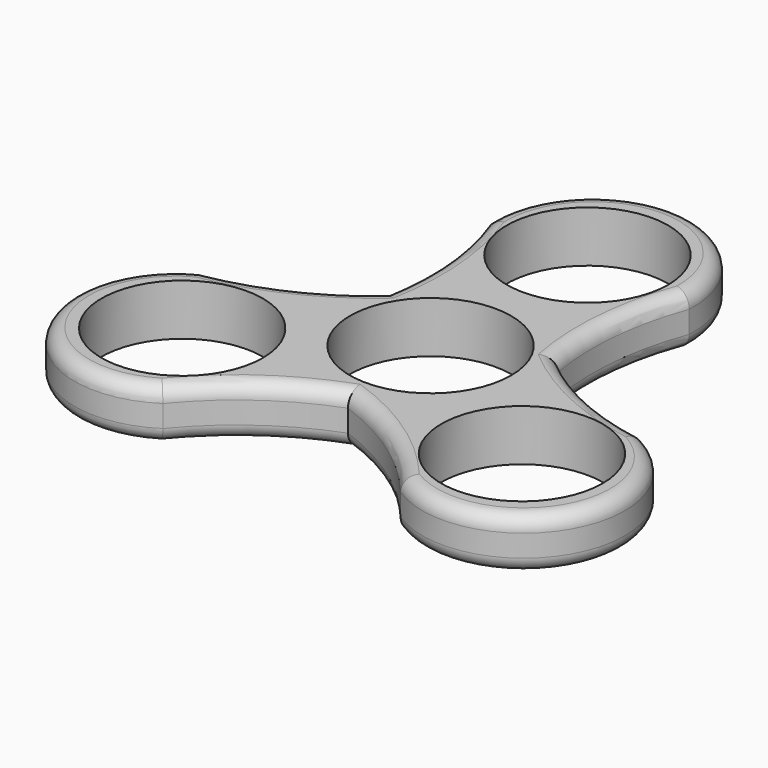
from build123d import *

# Parameters (mm, degrees)
F0_R         = 11
F1_DEPTH     = 7
F2_T3_ANGLE  = 45.2058743493
F2_S4_R      = 38
F2_T5_DEPTH  = 19
F2_T8_ANGLE  = 227.522654694
F2_T11_ANGLE = 45.8937746322
F2_S12_R     = 38
F2_T13_DEPTH = 20
F2_T16_ANGLE = 45.2058743493
F2_S17_R     = 38
F2_T18_DEPTH = 20
F2_T21_ANGLE = 227.522654694
F2_T24_ANGLE = 45.8937746322
F2_S25_R     = 38
F2_T26_DEPTH = 21
F2_T29_ANGLE = 45.2058743493
F2_S30_R     = 38
F2_T31_DEPTH = 21
F2_T34_ANGLE = 227.522654694
F2_T37_ANGLE = 45.8937746322
F2_S38_R     = 38
F2_T39_DEPTH = 20
F2_T43_ANGLE = 45.2058743493
F2_S44_R     = 38
F2_T45_DEPTH = 19
F2_T48_ANGLE = 45.8937746322
F2_S49_R     = 38
F2_T50_DEPTH = 20
F2_T55_ANGLE = 45.8937746322
F2_S56_R     = 38
F2_T57_DEPTH = 20
F2_T60_ANGLE = 45.2058743493
F2_S61_R     = 38
F2_T62_DEPTH = 20
F2_T67_ANGLE = 45.2058743493
F2_S68_R     = 38
F2_T69_DEPTH = 21
F2_T72_ANGLE = 45.8937746322
F2_S73_R     = 38
F2_T74_DEPTH = 21
F3_T3_ANGLE  = 227.522654694
F3_T6_ANGLE  = 45.2058743493
F3_S7_R      = 38
F3_T8_DEPTH  = 19
F3_T11_ANGLE = 45.8937746322
F3_S12_R     = 38
F3_T13_DEPTH = 20
F3_T16_ANGLE = 227.522654694
F3_T19_ANGLE = 45.2058743493
F3_S20_R     = 38
F3_T21_DEPTH = 21
F3_T24_ANGLE = 45.8937746322
F3_S25_R     = 38
F3_T26_DEPTH = 21
F3_T29_ANGLE = 227.522654694
F3_T32_ANGLE = 45.2058743493
F3_S33_R     = 38
F3_T34_DEPTH = 20
F3_T37_ANGLE = 45.8937746322
F3_S38_R     = 38
F3_T39_DEPTH = 20
F3_T43_ANGLE = 45.8937746322
F3_S44_R     = 38
F3_T45_DEPTH = 20
F3_T48_ANGLE = 45.2058743493
F3_S49_R     = 38
F3_T50_DEPTH = 19
F3_T55_ANGLE = 45.8937746322
F3_S56_R     = 38
F3_T57_DEPTH = 21
F3_T60_ANGLE = 45.2058743493
F3_S61_R     = 38
F3_T62_DEPTH = 21
F3_T67_ANGLE = 45.8937746322
F3_S68_R     = 38
F3_T69_DEPTH = 20
F3_T72_ANGLE = 45.2058743493
F3_S73_R     = 38
F3_T74_DEPTH = 20


# Not quite as in the source:
# - a fillet or chamfer that OpenCascade refuses, or shapes differently, is made with other operations: its cross-section is extruded or revolved along the edge and cut away or added


with BuildPart() as f1:
    # F0 (on Top) → F1 (new body)
    with BuildSketch(Plane.XY):
        with BuildLine():
            ThreePointArc((12.0468410067, 6.6555924166), (11.6038749685, 16.833912258), (13.8810481876, 26.764113456))
            ThreePointArc((13.8810481876, 26.764113456), (0.0907252543, 41.2909770134), (-13.6995976791, 26.764113456))
            ThreePointArc((-13.6995976791, 26.764113456), (-11.4438268991, 17.0610116136), (-11.7873326133, 7.1050741388))
            ThreePointArc((-11.7873326133, 7.1050741388), (-20.3805331447, 1.6322943761), (-30.1189262565, -1.3607163664))
            ThreePointArc((-30.1189262565, -1.3607163664), (-35.8043976678, -20.5669181317), (-16.3286033231, -25.2462563397))
            ThreePointArc((-16.3286033231, -25.2462563397), (-9.053356022, -18.4411506179), (-0.2595083933, -13.7606665554))
            ThreePointArc((-0.2595083933, -13.7606665554), (8.7766581762, -18.466206634), (16.2378780689, -25.4033970896))
            ThreePointArc((16.2378780689, -25.4033970896), (35.7136724135, -20.7240588817), (30.0282010022, -1.5178571163))
            ThreePointArc((30.0282010022, -1.5178571163), (20.4971829212, 1.3801390044), (12.0468410067, 6.6555924166))
        make_face()
        with Locations((-23.1784021627, -13.382056728)):
            Circle(F0_R, mode=Mode.SUBTRACT)
        with Locations((23.1784021627, -13.382056728)):
            Circle(F0_R, mode=Mode.SUBTRACT)
        Circle(F0_R, mode=Mode.SUBTRACT)
        with Locations((0, 26.764113456)):
            Circle(F0_R, mode=Mode.SUBTRACT)
    extrude(amount=F1_DEPTH)

    # F2: fillet of radius 2 on 9 edges, made by hand


with BuildPart() as f2_tool1:
    # F2_s2 → F2_t3 (revolve)
    with BuildSketch(Plane(origin=(-16.5393520653, 30.8992120032, 0), x_dir=(0, 0, 1), z_dir=(-0.4719154962, 0.8816437855, 0))):
        with BuildLine():
            ThreePointArc((5, 0.8807372995), (6.4142135624, 1.4665237371), (7, 2.8807372995))
            Line((7, 2.8807372995), (7, 0.8807372995))
            Line((7, 0.8807372995), (5, 0.8807372995))
        make_face()
    revolve(axis=Axis((-49.2653193466, 13.382056728, 7), (0, 0, -1)), revolution_arc=F2_T3_ANGLE)

    # F2_s4 → F2_t5 (intersect, symmetric)
    with BuildSketch(Plane.XY.offset(5.3)):
        with Locations((-36.3125860089, 36.1311304656)):
            Circle(F2_S4_R)
    extrude(amount=F2_T5_DEPTH, both=True, mode=Mode.INTERSECT)


with BuildPart() as f2_tool6:
    # F2_s7 → F2_t8 (revolve)
    with BuildSketch(Plane(origin=(10.1493203818, 23.0537204739, 0), x_dir=(0, 0, 1), z_dir=(-0.4029276386, -0.9152318384, 0))):
        with BuildLine():
            ThreePointArc((5, -2.8187794742), (6.4142135624, -2.2329930365), (7, -0.8187794742))
            Line((7, -0.8187794742), (7, -2.8187794742))
            Line((7, -2.8187794742), (5, -2.8187794742))
        make_face()
    revolve(axis=Axis((0.0907252543, 27.4819820491, 7), (0, 0, 1)), revolution_arc=F2_T8_ANGLE)


with BuildPart() as f2_tool9:
    # F2_s10 → F2_t11 (revolve)
    with BuildSketch(Plane(origin=(0.7055478119, -2.2061129258, 0), x_dir=(0, 0, 1), z_dir=(0.3046158068, -0.9524753069, 0))):
        with BuildLine():
            ThreePointArc((5, -13.1732132997), (6.4142135624, -12.5874268621), (7, -11.1732132997))
            Line((7, -11.1732132997), (7, -13.1732132997))
            Line((7, -13.1732132997), (5, -13.1732132997))
        make_face()
    revolve(axis=Axis((49.4467698551, 13.382056728, 7), (0, 0, -1)), revolution_arc=F2_T11_ANGLE)

    # F2_s12 → F2_t13 (intersect, symmetric)
    with BuildSketch(Plane.XY.offset(5.3)):
        with Locations((36.2218607546, 35.9739897157)):
            Circle(F2_S12_R)
    extrude(amount=F2_T13_DEPTH, both=True, mode=Mode.INTERSECT)


with BuildPart() as f2_tool14:
    # F2_s15 → F2_t16 (revolve)
    with BuildSketch(Plane(origin=(35.0291785844, -1.1261069509, 0), x_dir=(0, 0, 1), z_dir=(0.9994836634, -0.0321310846, 0))):
        with BuildLine():
            ThreePointArc((5, 0.8807372995), (6.4142135624, 1.4665237371), (7, 2.8807372995))
            Line((7, 2.8807372995), (7, 0.8807372995))
            Line((7, 0.8807372995), (5, 0.8807372995))
        make_face()
    revolve(axis=Axis((36.2218607546, 35.9739897157, 7), (0, 0, -1)), revolution_arc=F2_T16_ANGLE)

    # F2_s17 → F2_t18 (intersect, symmetric)
    with BuildSketch(Plane.XY.offset(5.3)):
        with Locations((49.4467698551, 13.382056728)):
            Circle(F2_S17_R)
    extrude(amount=F2_T18_DEPTH, both=True, mode=Mode.INTERSECT)


with BuildPart() as f2_tool19:
    # F2_s20 → F2_t21 (revolve)
    with BuildSketch(Plane(origin=(14.8904473912, -20.3164295188, 0), x_dir=(0, 0, 1), z_dir=(-0.5911502031, 0.8065614901, 0))):
        with BuildLine():
            ThreePointArc((5, -2.8187794742), (6.4142135624, -2.2329930365), (7, -0.8187794742))
            Line((7, -0.8187794742), (7, -2.8187794742))
            Line((7, -2.8187794742), (5, -2.8187794742))
        make_face()
    revolve(axis=Axis((23.7547319738, -13.8195613995, 7), (0, 0, 1)), revolution_arc=F2_T21_ANGLE)


with BuildPart() as f2_tool22:
    # F2_s23 → F2_t24 (revolve)
    with BuildSketch(Plane(origin=(-2.2633237433, 0.4920341342, 0), x_dir=(0, 0, 1), z_dir=(-0.9771757156, 0.2124326264, 0))):
        with BuildLine():
            ThreePointArc((5, -13.1732132997), (6.4142135624, -12.5874268621), (7, -11.1732132997))
            Line((7, -11.1732132997), (7, -13.1732132997))
            Line((7, -13.1732132997), (5, -13.1732132997))
        make_face()
    revolve(axis=Axis((-13.1341838462, -49.5131871936, 7), (0, 0, -1)), revolution_arc=F2_T24_ANGLE)

    # F2_s25 → F2_t26 (intersect, symmetric)
    with BuildSketch(Plane.XY.offset(5.3)):
        with Locations((13.0434585919, -49.3560464437)):
            Circle(F2_S25_R)
    extrude(amount=F2_T26_DEPTH, both=True, mode=Mode.INTERSECT)


with BuildPart() as f2_tool27:
    # F2_s28 → F2_t29 (revolve)
    with BuildSketch(Plane(origin=(-18.4898265191, -29.7731050523, 0), x_dir=(0, 0, 1), z_dir=(-0.5275681672, -0.8495127009, 0))):
        with BuildLine():
            ThreePointArc((5, 0.8807372995), (6.4142135624, 1.4665237371), (7, 2.8807372995))
            Line((7, 2.8807372995), (7, 0.8807372995))
            Line((7, 0.8807372995), (5, 0.8807372995))
        make_face()
    revolve(axis=Axis((13.0434585919, -49.3560464437, 7), (0, 0, -1)), revolution_arc=F2_T29_ANGLE)

    # F2_s30 → F2_t31 (intersect, symmetric)
    with BuildSketch(Plane.XY.offset(5.3)):
        with Locations((-13.1341838462, -49.5131871936)):
            Circle(F2_S30_R)
    extrude(amount=F2_T31_DEPTH, both=True, mode=Mode.INTERSECT)


with BuildPart() as f2_tool32:
    # F2_s33 → F2_t34 (revolve)
    with BuildSketch(Plane(origin=(-25.0397677731, -2.7372909551, 0), x_dir=(0, 0, 1), z_dir=(0.9940778417, 0.1086703483, 0))):
        with BuildLine():
            ThreePointArc((5, -2.8187794742), (6.4142135624, -2.2329930365), (7, -0.8187794742))
            Line((7, -0.8187794742), (7, -2.8187794742))
            Line((7, -2.8187794742), (5, -2.8187794742))
        make_face()
    revolve(axis=Axis((-23.845457228, -13.6624206496, 7), (0, 0, 1)), revolution_arc=F2_T34_ANGLE)


with BuildPart() as f2_tool35:
    # F2_s36 → F2_t37 (revolve)
    with BuildSketch(Plane(origin=(1.5577759314, 1.7140787916, 0), x_dir=(0, 0, 1), z_dir=(0.6725599089, 0.7400426805, 0))):
        with BuildLine():
            ThreePointArc((5, -13.1732132997), (6.4142135624, -12.5874268621), (7, -11.1732132997))
            Line((7, -11.1732132997), (7, -13.1732132997))
            Line((7, -13.1732132997), (5, -13.1732132997))
        make_face()
    revolve(axis=Axis((-36.3125860089, 36.1311304656, 7), (0, 0, -1)), revolution_arc=F2_T37_ANGLE)

    # F2_s38 → F2_t39 (intersect, symmetric)
    with BuildSketch(Plane.XY.offset(6)):
        with Locations((-49.2653193466, 13.382056728)):
            Circle(F2_S38_R)
    extrude(amount=F2_T39_DEPTH, both=True, mode=Mode.INTERSECT)


with BuildPart() as f2_tool41:
    # F2_s42 → F2_t43 (revolve)
    with BuildSketch(Plane(origin=(-16.5393520653, 30.8992120032, 0), x_dir=(0, 0, 1), z_dir=(-0.4719154962, 0.8816437855, 0))):
        with BuildLine():
            ThreePointArc((5, 0.8807372995), (6.4142135624, 1.4665237371), (7, 2.8807372995))
            Line((7, 2.8807372995), (7, 0.8807372995))
            Line((7, 0.8807372995), (5, 0.8807372995))
        make_face()
    revolve(axis=Axis((-49.2653193466, 13.382056728, 7), (0, 0, -1)), revolution_arc=F2_T43_ANGLE)

    # F2_s44 → F2_t45 (cut, symmetric)
    with BuildSketch(Plane.XY.offset(5.3)):
        with Locations((-36.3125860089, 36.1311304656)):
            Circle(F2_S44_R)
    extrude(amount=F2_T45_DEPTH, both=True, mode=Mode.SUBTRACT)


with BuildPart() as f2_tool46:
    # F2_s47 → F2_t48 (revolve)
    with BuildSketch(Plane(origin=(1.5577759314, 1.7140787916, 0), x_dir=(0, 0, 1), z_dir=(0.6725599089, 0.7400426805, 0))):
        with BuildLine():
            ThreePointArc((5, -13.1732132997), (6.4142135624, -12.5874268621), (7, -11.1732132997))
            Line((7, -11.1732132997), (7, -13.1732132997))
            Line((7, -13.1732132997), (5, -13.1732132997))
        make_face()
    revolve(axis=Axis((-36.3125860089, 36.1311304656, 7), (0, 0, -1)), revolution_arc=F2_T48_ANGLE)

    # F2_s49 → F2_t50 (cut, symmetric)
    with BuildSketch(Plane.XY.offset(6)):
        with Locations((-49.2653193466, 13.382056728)):
            Circle(F2_S49_R)
    extrude(amount=F2_T50_DEPTH, both=True, mode=Mode.SUBTRACT)


with BuildPart() as f2_tool41_1:
    add(f2_tool41.part)

    # F2_t51: intersect F2_tool46
    add(f2_tool46.part, mode=Mode.INTERSECT)


with BuildPart() as f2_tool53:
    # F2_s54 → F2_t55 (revolve)
    with BuildSketch(Plane(origin=(0.7055478119, -2.2061129258, 0), x_dir=(0, 0, 1), z_dir=(0.3046158068, -0.9524753069, 0))):
        with BuildLine():
            ThreePointArc((5, -13.1732132997), (6.4142135624, -12.5874268621), (7, -11.1732132997))
            Line((7, -11.1732132997), (7, -13.1732132997))
            Line((7, -13.1732132997), (5, -13.1732132997))
        make_face()
    revolve(axis=Axis((49.4467698551, 13.382056728, 7), (0, 0, -1)), revolution_arc=F2_T55_ANGLE)

    # F2_s56 → F2_t57 (cut, symmetric)
    with BuildSketch(Plane.XY.offset(5.3)):
        with Locations((36.2218607546, 35.9739897157)):
            Circle(F2_S56_R)
    extrude(amount=F2_T57_DEPTH, both=True, mode=Mode.SUBTRACT)


with BuildPart() as f2_tool58:
    # F2_s59 → F2_t60 (revolve)
    with BuildSketch(Plane(origin=(35.0291785844, -1.1261069509, 0), x_dir=(0, 0, 1), z_dir=(0.9994836634, -0.0321310846, 0))):
        with BuildLine():
            ThreePointArc((5, 0.8807372995), (6.4142135624, 1.4665237371), (7, 2.8807372995))
            Line((7, 2.8807372995), (7, 0.8807372995))
            Line((7, 0.8807372995), (5, 0.8807372995))
        make_face()
    revolve(axis=Axis((36.2218607546, 35.9739897157, 7), (0, 0, -1)), revolution_arc=F2_T60_ANGLE)

    # F2_s61 → F2_t62 (cut, symmetric)
    with BuildSketch(Plane.XY.offset(5.3)):
        with Locations((49.4467698551, 13.382056728)):
            Circle(F2_S61_R)
    extrude(amount=F2_T62_DEPTH, both=True, mode=Mode.SUBTRACT)


with BuildPart() as f2_tool53_1:
    add(f2_tool53.part)

    # F2_t63: intersect F2_tool58
    add(f2_tool58.part, mode=Mode.INTERSECT)


with BuildPart() as f2_tool65:
    # F2_s66 → F2_t67 (revolve)
    with BuildSketch(Plane(origin=(-18.4898265191, -29.7731050523, 0), x_dir=(0, 0, 1), z_dir=(-0.5275681672, -0.8495127009, 0))):
        with BuildLine():
            ThreePointArc((5, 0.8807372995), (6.4142135624, 1.4665237371), (7, 2.8807372995))
            Line((7, 2.8807372995), (7, 0.8807372995))
            Line((7, 0.8807372995), (5, 0.8807372995))
        make_face()
    revolve(axis=Axis((13.0434585919, -49.3560464437, 7), (0, 0, -1)), revolution_arc=F2_T67_ANGLE)

    # F2_s68 → F2_t69 (cut, symmetric)
    with BuildSketch(Plane.XY.offset(5.3)):
        with Locations((-13.1341838462, -49.5131871936)):
            Circle(F2_S68_R)
    extrude(amount=F2_T69_DEPTH, both=True, mode=Mode.SUBTRACT)


with BuildPart() as f2_tool70:
    # F2_s71 → F2_t72 (revolve)
    with BuildSketch(Plane(origin=(-2.2633237433, 0.4920341342, 0), x_dir=(0, 0, 1), z_dir=(-0.9771757156, 0.2124326264, 0))):
        with BuildLine():
            ThreePointArc((5, -13.1732132997), (6.4142135624, -12.5874268621), (7, -11.1732132997))
            Line((7, -11.1732132997), (7, -13.1732132997))
            Line((7, -13.1732132997), (5, -13.1732132997))
        make_face()
    revolve(axis=Axis((-13.1341838462, -49.5131871936, 7), (0, 0, -1)), revolution_arc=F2_T72_ANGLE)

    # F2_s73 → F2_t74 (cut, symmetric)
    with BuildSketch(Plane.XY.offset(5.3)):
        with Locations((13.0434585919, -49.3560464437)):
            Circle(F2_S73_R)
    extrude(amount=F2_T74_DEPTH, both=True, mode=Mode.SUBTRACT)


with BuildPart() as f2_tool65_1:
    add(f2_tool65.part)

    # F2_t75: intersect F2_tool70
    add(f2_tool70.part, mode=Mode.INTERSECT)


with BuildPart() as f1_1:
    add(f1.part)

    # F2_t76: cut F2_tool1, F2_tool6, F2_tool9, F2_tool14, F2_tool19, F2_tool22, F2_tool27, F2_tool32, F2_tool35, F2_tool41, F2_tool53, F2_tool65
    add([f2_tool1.part, f2_tool6.part, f2_tool9.part, f2_tool14.part, f2_tool19.part, f2_tool22.part, f2_tool27.part, f2_tool32.part, f2_tool35.part, f2_tool41_1.part, f2_tool53_1.part, f2_tool65_1.part], mode=Mode.SUBTRACT)

    # F3: fillet of radius 2 on 9 edges, made by hand


with BuildPart() as f3_tool1:
    # F3_s2 → F3_t3 (revolve)
    with BuildSketch(Plane(origin=(10.1493203818, 23.0537204739, 0), x_dir=(0, 0, 1), z_dir=(-0.4029276386, -0.9152318384, 0))):
        with BuildLine():
            ThreePointArc((2, -2.8187794742), (0.5857864376, -2.2329930365), (0, -0.8187794742))
            Line((0, -0.8187794742), (0, -2.8187794742))
            Line((0, -2.8187794742), (2, -2.8187794742))
        make_face()
    revolve(axis=Axis((0.0907252543, 27.4819820491, 0), (0, 0, 1)), revolution_arc=F3_T3_ANGLE)


with BuildPart() as f3_tool4:
    # F3_s5 → F3_t6 (revolve)
    with BuildSketch(Plane(origin=(-16.5393520653, 30.8992120032, 0), x_dir=(0, 0, 1), z_dir=(-0.4719154962, 0.8816437855, 0))):
        with BuildLine():
            ThreePointArc((2, 0.8807372995), (0.5857864376, 1.4665237371), (0, 2.8807372995))
            Line((0, 2.8807372995), (0, 0.8807372995))
            Line((0, 0.8807372995), (2, 0.8807372995))
        make_face()
    revolve(axis=Axis((-49.2653193466, 13.382056728, 0), (0, 0, -1)), revolution_arc=F3_T6_ANGLE)

    # F3_s7 → F3_t8 (intersect, symmetric)
    with BuildSketch(Plane.XY.offset(1.7)):
        with Locations((-36.3125860089, 36.1311304656)):
            Circle(F3_S7_R)
    extrude(amount=F3_T8_DEPTH, both=True, mode=Mode.INTERSECT)


with BuildPart() as f3_tool9:
    # F3_s10 → F3_t11 (revolve)
    with BuildSketch(Plane(origin=(1.5577759314, 1.7140787916, 0), x_dir=(0, 0, 1), z_dir=(0.6725599089, 0.7400426805, 0))):
        with BuildLine():
            ThreePointArc((2, -13.1732132997), (0.5857864376, -12.5874268621), (0, -11.1732132997))
            Line((0, -11.1732132997), (0, -13.1732132997))
            Line((0, -13.1732132997), (2, -13.1732132997))
        make_face()
    revolve(axis=Axis((-36.3125860089, 36.1311304656, 0), (0, 0, -1)), revolution_arc=F3_T11_ANGLE)

    # F3_s12 → F3_t13 (intersect, symmetric)
    with BuildSketch(Plane.XY.offset(1)):
        with Locations((-49.2653193466, 13.382056728)):
            Circle(F3_S12_R)
    extrude(amount=F3_T13_DEPTH, both=True, mode=Mode.INTERSECT)


with BuildPart() as f3_tool14:
    # F3_s15 → F3_t16 (revolve)
    with BuildSketch(Plane(origin=(-25.0397677731, -2.7372909551, 0), x_dir=(0, 0, 1), z_dir=(0.9940778417, 0.1086703483, 0))):
        with BuildLine():
            ThreePointArc((2, -2.8187794742), (0.5857864376, -2.2329930365), (0, -0.8187794742))
            Line((0, -0.8187794742), (0, -2.8187794742))
            Line((0, -2.8187794742), (2, -2.8187794742))
        make_face()
    revolve(axis=Axis((-23.845457228, -13.6624206496, 0), (0, 0, 1)), revolution_arc=F3_T16_ANGLE)


with BuildPart() as f3_tool17:
    # F3_s18 → F3_t19 (revolve)
    with BuildSketch(Plane(origin=(-18.4898265191, -29.7731050523, 0), x_dir=(0, 0, 1), z_dir=(-0.5275681672, -0.8495127009, 0))):
        with BuildLine():
            ThreePointArc((2, 0.8807372995), (0.5857864376, 1.4665237371), (0, 2.8807372995))
            Line((0, 2.8807372995), (0, 0.8807372995))
            Line((0, 0.8807372995), (2, 0.8807372995))
        make_face()
    revolve(axis=Axis((13.0434585919, -49.3560464437, 0), (0, 0, -1)), revolution_arc=F3_T19_ANGLE)

    # F3_s20 → F3_t21 (intersect, symmetric)
    with BuildSketch(Plane.XY.offset(1.7)):
        with Locations((-13.1341838462, -49.5131871936)):
            Circle(F3_S20_R)
    extrude(amount=F3_T21_DEPTH, both=True, mode=Mode.INTERSECT)


with BuildPart() as f3_tool22:
    # F3_s23 → F3_t24 (revolve)
    with BuildSketch(Plane(origin=(-2.2633237433, 0.4920341342, 0), x_dir=(0, 0, 1), z_dir=(-0.9771757156, 0.2124326264, 0))):
        with BuildLine():
            ThreePointArc((2, -13.1732132997), (0.5857864376, -12.5874268621), (0, -11.1732132997))
            Line((0, -11.1732132997), (0, -13.1732132997))
            Line((0, -13.1732132997), (2, -13.1732132997))
        make_face()
    revolve(axis=Axis((-13.1341838462, -49.5131871936, 0), (0, 0, -1)), revolution_arc=F3_T24_ANGLE)

    # F3_s25 → F3_t26 (intersect, symmetric)
    with BuildSketch(Plane.XY.offset(1.7)):
        with Locations((13.0434585919, -49.3560464437)):
            Circle(F3_S25_R)
    extrude(amount=F3_T26_DEPTH, both=True, mode=Mode.INTERSECT)


with BuildPart() as f3_tool27:
    # F3_s28 → F3_t29 (revolve)
    with BuildSketch(Plane(origin=(14.8904473912, -20.3164295188, 0), x_dir=(0, 0, 1), z_dir=(-0.5911502031, 0.8065614901, 0))):
        with BuildLine():
            ThreePointArc((2, -2.8187794742), (0.5857864376, -2.2329930365), (0, -0.8187794742))
            Line((0, -0.8187794742), (0, -2.8187794742))
            Line((0, -2.8187794742), (2, -2.8187794742))
        make_face()
    revolve(axis=Axis((23.7547319738, -13.8195613995, 0), (0, 0, 1)), revolution_arc=F3_T29_ANGLE)


with BuildPart() as f3_tool30:
    # F3_s31 → F3_t32 (revolve)
    with BuildSketch(Plane(origin=(35.0291785844, -1.1261069509, 0), x_dir=(0, 0, 1), z_dir=(0.9994836634, -0.0321310846, 0))):
        with BuildLine():
            ThreePointArc((2, 0.8807372995), (0.5857864376, 1.4665237371), (0, 2.8807372995))
            Line((0, 2.8807372995), (0, 0.8807372995))
            Line((0, 0.8807372995), (2, 0.8807372995))
        make_face()
    revolve(axis=Axis((36.2218607546, 35.9739897157, 0), (0, 0, -1)), revolution_arc=F3_T32_ANGLE)

    # F3_s33 → F3_t34 (intersect, symmetric)
    with BuildSketch(Plane.XY.offset(1.7)):
        with Locations((49.4467698551, 13.382056728)):
            Circle(F3_S33_R)
    extrude(amount=F3_T34_DEPTH, both=True, mode=Mode.INTERSECT)


with BuildPart() as f3_tool35:
    # F3_s36 → F3_t37 (revolve)
    with BuildSketch(Plane(origin=(0.7055478119, -2.2061129258, 0), x_dir=(0, 0, 1), z_dir=(0.3046158068, -0.9524753069, 0))):
        with BuildLine():
            ThreePointArc((2, -13.1732132997), (0.5857864376, -12.5874268621), (0, -11.1732132997))
            Line((0, -11.1732132997), (0, -13.1732132997))
            Line((0, -13.1732132997), (2, -13.1732132997))
        make_face()
    revolve(axis=Axis((49.4467698551, 13.382056728, 0), (0, 0, -1)), revolution_arc=F3_T37_ANGLE)

    # F3_s38 → F3_t39 (intersect, symmetric)
    with BuildSketch(Plane.XY.offset(1.7)):
        with Locations((36.2218607546, 35.9739897157)):
            Circle(F3_S38_R)
    extrude(amount=F3_T39_DEPTH, both=True, mode=Mode.INTERSECT)


with BuildPart() as f3_tool41:
    # F3_s42 → F3_t43 (revolve)
    with BuildSketch(Plane(origin=(1.5577759314, 1.7140787916, 0), x_dir=(0, 0, 1), z_dir=(0.6725599089, 0.7400426805, 0))):
        with BuildLine():
            ThreePointArc((2, -13.1732132997), (0.5857864376, -12.5874268621), (0, -11.1732132997))
            Line((0, -11.1732132997), (0, -13.1732132997))
            Line((0, -13.1732132997), (2, -13.1732132997))
        make_face()
    revolve(axis=Axis((-36.3125860089, 36.1311304656, 0), (0, 0, -1)), revolution_arc=F3_T43_ANGLE)

    # F3_s44 → F3_t45 (cut, symmetric)
    with BuildSketch(Plane.XY.offset(1)):
        with Locations((-49.2653193466, 13.382056728)):
            Circle(F3_S44_R)
    extrude(amount=F3_T45_DEPTH, both=True, mode=Mode.SUBTRACT)


with BuildPart() as f3_tool46:
    # F3_s47 → F3_t48 (revolve)
    with BuildSketch(Plane(origin=(-16.5393520653, 30.8992120032, 0), x_dir=(0, 0, 1), z_dir=(-0.4719154962, 0.8816437855, 0))):
        with BuildLine():
            ThreePointArc((2, 0.8807372995), (0.5857864376, 1.4665237371), (0, 2.8807372995))
            Line((0, 2.8807372995), (0, 0.8807372995))
            Line((0, 0.8807372995), (2, 0.8807372995))
        make_face()
    revolve(axis=Axis((-49.2653193466, 13.382056728, 0), (0, 0, -1)), revolution_arc=F3_T48_ANGLE)

    # F3_s49 → F3_t50 (cut, symmetric)
    with BuildSketch(Plane.XY.offset(1.7)):
        with Locations((-36.3125860089, 36.1311304656)):
            Circle(F3_S49_R)
    extrude(amount=F3_T50_DEPTH, both=True, mode=Mode.SUBTRACT)


with BuildPart() as f3_tool41_1:
    add(f3_tool41.part)

    # F3_t51: intersect F3_tool46
    add(f3_tool46.part, mode=Mode.INTERSECT)


with BuildPart() as f3_tool53:
    # F3_s54 → F3_t55 (revolve)
    with BuildSketch(Plane(origin=(-2.2633237433, 0.4920341342, 0), x_dir=(0, 0, 1), z_dir=(-0.9771757156, 0.2124326264, 0))):
        with BuildLine():
            ThreePointArc((2, -13.1732132997), (0.5857864376, -12.5874268621), (0, -11.1732132997))
            Line((0, -11.1732132997), (0, -13.1732132997))
            Line((0, -13.1732132997), (2, -13.1732132997))
        make_face()
    revolve(axis=Axis((-13.1341838462, -49.5131871936, 0), (0, 0, -1)), revolution_arc=F3_T55_ANGLE)

    # F3_s56 → F3_t57 (cut, symmetric)
    with BuildSketch(Plane.XY.offset(1.7)):
        with Locations((13.0434585919, -49.3560464437)):
            Circle(F3_S56_R)
    extrude(amount=F3_T57_DEPTH, both=True, mode=Mode.SUBTRACT)


with BuildPart() as f3_tool58:
    # F3_s59 → F3_t60 (revolve)
    with BuildSketch(Plane(origin=(-18.4898265191, -29.7731050523, 0), x_dir=(0, 0, 1), z_dir=(-0.5275681672, -0.8495127009, 0))):
        with BuildLine():
            ThreePointArc((2, 0.8807372995), (0.5857864376, 1.4665237371), (0, 2.8807372995))
            Line((0, 2.8807372995), (0, 0.8807372995))
            Line((0, 0.8807372995), (2, 0.8807372995))
        make_face()
    revolve(axis=Axis((13.0434585919, -49.3560464437, 0), (0, 0, -1)), revolution_arc=F3_T60_ANGLE)

    # F3_s61 → F3_t62 (cut, symmetric)
    with BuildSketch(Plane.XY.offset(1.7)):
        with Locations((-13.1341838462, -49.5131871936)):
            Circle(F3_S61_R)
    extrude(amount=F3_T62_DEPTH, both=True, mode=Mode.SUBTRACT)


with BuildPart() as f3_tool53_1:
    add(f3_tool53.part)

    # F3_t63: intersect F3_tool58
    add(f3_tool58.part, mode=Mode.INTERSECT)


with BuildPart() as f3_tool65:
    # F3_s66 → F3_t67 (revolve)
    with BuildSketch(Plane(origin=(0.7055478119, -2.2061129258, 0), x_dir=(0, 0, 1), z_dir=(0.3046158068, -0.9524753069, 0))):
        with BuildLine():
            ThreePointArc((2, -13.1732132997), (0.5857864376, -12.5874268621), (0, -11.1732132997))
            Line((0, -11.1732132997), (0, -13.1732132997))
            Line((0, -13.1732132997), (2, -13.1732132997))
        make_face()
    revolve(axis=Axis((49.4467698551, 13.382056728, 0), (0, 0, -1)), revolution_arc=F3_T67_ANGLE)

    # F3_s68 → F3_t69 (cut, symmetric)
    with BuildSketch(Plane.XY.offset(1.7)):
        with Locations((36.2218607546, 35.9739897157)):
            Circle(F3_S68_R)
    extrude(amount=F3_T69_DEPTH, both=True, mode=Mode.SUBTRACT)


with BuildPart() as f3_tool70:
    # F3_s71 → F3_t72 (revolve)
    with BuildSketch(Plane(origin=(35.0291785844, -1.1261069509, 0), x_dir=(0, 0, 1), z_dir=(0.9994836634, -0.0321310846, 0))):
        with BuildLine():
            ThreePointArc((2, 0.8807372995), (0.5857864376, 1.4665237371), (0, 2.8807372995))
            Line((0, 2.8807372995), (0, 0.8807372995))
            Line((0, 0.8807372995), (2, 0.8807372995))
        make_face()
    revolve(axis=Axis((36.2218607546, 35.9739897157, 0), (0, 0, -1)), revolution_arc=F3_T72_ANGLE)

    # F3_s73 → F3_t74 (cut, symmetric)
    with BuildSketch(Plane.XY.offset(1.7)):
        with Locations((49.4467698551, 13.382056728)):
            Circle(F3_S73_R)
    extrude(amount=F3_T74_DEPTH, both=True, mode=Mode.SUBTRACT)


with BuildPart() as f3_tool65_1:
    add(f3_tool65.part)

    # F3_t75: intersect F3_tool70
    add(f3_tool70.part, mode=Mode.INTERSECT)


with BuildPart() as f1_2:
    add(f1_1.part)

    # F3_t76: cut F3_tool1, F3_tool4, F3_tool9, F3_tool14, F3_tool17, F3_tool22, F3_tool27, F3_tool30, F3_tool35, F3_tool41, F3_tool53, F3_tool65
    add([f3_tool1.part, f3_tool4.part, f3_tool9.part, f3_tool14.part, f3_tool17.part, f3_tool22.part, f3_tool27.part, f3_tool30.part, f3_tool35.part, f3_tool41_1.part, f3_tool53_1.part, f3_tool65_1.part], mode=Mode.SUBTRACT)


solid = f1_2.part
